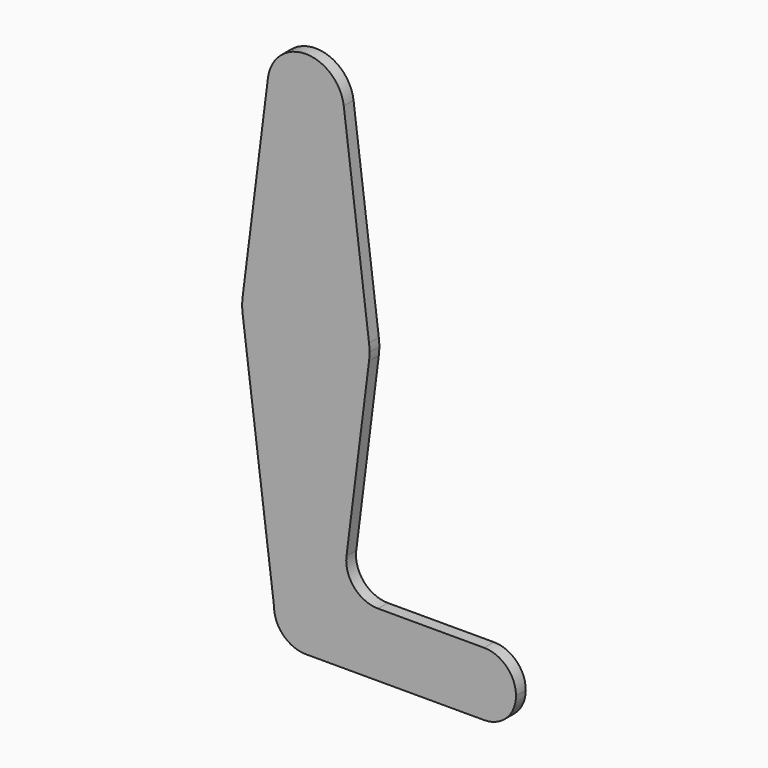
from build123d import *

# Parameters (mm, degrees)
F0_R     = 3.175
F1_DEPTH = 3.048


# Not quite as in the source:
# - ends of sketch curves that miss each other by under 0.0002 mm in the source are joined


with BuildPart() as f1:
    # F0 (on Front) → F1 (new body)
    with BuildSketch(Plane.XZ):
        with BuildLine():
            ThreePointArc((-7.9375, 0), (0, 7.9375), (7.9375, 0))
            ThreePointArc((7.9375, 0), (5.6126600757, -5.6126600757), (0, -7.9375))
            Line((0, -7.9375), (44.45, -7.9375))
            ThreePointArc((44.45, -7.9375), (36.5125, 0), (44.45, 7.9375))
            Line((44.45, 7.9375), (18.0149584735, 7.9375))
            ThreePointArc((18.0149584735, 7.9375), (12.0523084735, 10.6291369817), (10.127113946, 16.881475))
            Line((10.127113946, 16.881475), (15.7504882737, 61.515625))
            ThreePointArc((15.7504882737, 61.515625), (15.8438414904, 62.5058612634), (15.875, 63.5))
            ThreePointArc((15.875, 63.5), (15.8438414904, 64.4941387366), (15.7504882737, 65.484375))
            ThreePointArc((15.7504882737, 65.484375), (0, 79.375), (-15.7504882737, 65.484375))
            ThreePointArc((-15.7504882737, 65.484375), (-15.875, 63.4999684915), (-15.7504803964, 61.5155624772))
            Line((-15.7504803964, 61.5155624772), (-7.9375, 0))
        make_face()
        with Locations((0, 63.5)):
            Circle(F0_R, mode=Mode.SUBTRACT)
        with BuildLine():
            Line((-9.4502929642, 115.490625), (-15.7504882737, 65.484375))
            ThreePointArc((-15.7504882737, 65.484375), (0, 79.375), (15.7504882737, 65.484375))
            Line((15.7504882737, 65.484375), (9.4502929642, 115.490625))
            ThreePointArc((9.4502929642, 115.490625), (9.5063048942, 114.896483242), (9.525, 114.3))
            ThreePointArc((9.525, 114.3), (-0.596483242, 104.7936951058), (-9.4502929642, 115.490625))
        make_face()
        with Locations((-3.175, 100.0252)):
            Circle(F0_R, mode=Mode.SUBTRACT)
        with BuildLine():
            ThreePointArc((9.4502929642, 115.490625), (0, 123.825), (-9.4502929642, 115.490625))
            ThreePointArc((-9.4502929642, 115.490625), (-0.596483242, 104.7936951058), (9.525, 114.3))
            ThreePointArc((9.525, 114.3), (9.5063048942, 114.896483242), (9.4502929642, 115.490625))
        make_face()
        with Locations((0, 114.3)):
            Circle(F0_R, mode=Mode.SUBTRACT)
        with BuildLine():
            ThreePointArc((0, -7.9375), (5.6126600757, -5.6126600757), (7.9375, 0))
            ThreePointArc((7.9375, 0), (0, 7.9375), (-7.9375, 0))
            ThreePointArc((-7.9375, 0), (-5.6126600757, -5.6126600757), (0, -7.9375))
        make_face()
        Circle(F0_R, mode=Mode.SUBTRACT)
        with BuildLine():
            ThreePointArc((44.45, 7.9375), (36.5125, 0), (44.45, -7.9375))
            ThreePointArc((44.45, -7.9375), (50.0626600757, -5.6126600757), (52.3875, 0))
            ThreePointArc((52.3875, 0), (50.0626600757, 5.6126600757), (44.45, 7.9375))
        make_face()
        with Locations((44.45, 0)):
            Circle(F0_R, mode=Mode.SUBTRACT)
        with Locations((44.45, 0)):
            Circle(F0_R)
        with Locations((0, 63.5)):
            Circle(F0_R)
        with Locations((-3.175, 100.0252)):
            Circle(F0_R)
        with Locations((0, 114.3)):
            Circle(F0_R)
        Circle(F0_R)
    extrude(amount=F1_DEPTH)


solid = f1.part
